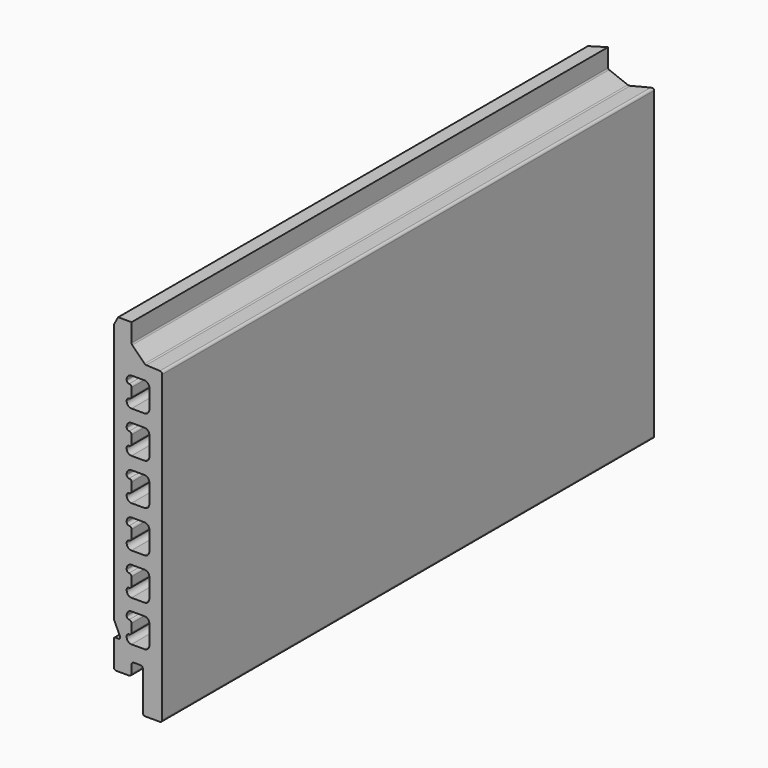
from build123d import *

# Parameters (mm, degrees)
F1_DEPTH      = 381
F3_DEPTH      = 711.2
F5_DEPTH      = 106.0997464
F5_DEPTH_BACK = 106.0997464


# Not quite as in the source:
# - ends of sketch curves that miss each other by under 0.0002 mm in the source are joined


with BuildPart() as f1:
    # F0 (on Front) → F1 (new body)
    with BuildSketch(Plane.XZ):
        with BuildLine():
            ThreePointArc((-14.9999680608, -58.9985104), (-14.96444377, -59.322873513), (-14.8595551032, -59.6318585804))
            Line((-14.8595551032, -59.6318585804), (-11.0988328608, -67.6967912))
            ThreePointArc((-11.0988328608, -67.6967912), (-11.1617050028, -68.655791158), (-12.004294, -69.1180454046))
            Line((-12.004294, -69.1180454046), (-14.0009118, -69.1180736))
            ThreePointArc((-14.0009118, -69.1180736), (-14.707352628, -69.410690972), (-14.99997, -70.1171318))
            Line((-14.99997, -70.1171318), (-14.99997, -85.599397))
            ThreePointArc((-14.99997, -85.599397), (-14.5606310505, -86.6600550505), (-13.499973, -87.099394))
            Line((-13.499973, -87.099394), (-5.5003446, -87.099394))
            ThreePointArc((-5.5003446, -87.099394), (-4.4396865495, -86.6600550505), (-4.0003476, -85.599397))
            Line((-4.0003476, -85.599397), (-4.0003476, -80.5996356))
            ThreePointArc((-4.0003476, -80.5996356), (-3.5610086505, -79.5389775495), (-2.5003506, -79.0996386))
            Line((-2.5003506, -79.0996386), (1.4838426, -79.0996386))
            ThreePointArc((1.4838426, -79.0996386), (2.5445365709, -79.5390134712), (2.9838395966, -80.5997372))
            Line((2.9838395966, -80.5997372), (2.98196, -104.5986224))
            ThreePointArc((2.98196, -104.5986224), (3.4212540492, -105.6593625482), (4.481957, -106.0987464))
            Line((4.481957, -106.0987464), (13.499973, -106.0987464))
            ThreePointArc((13.499973, -106.0987464), (14.5606310505, -105.6594074505), (14.99997, -104.5987494))
            Line((14.99997, -104.5987494), (14.99997, 83.7761342))
            ThreePointArc((14.99997, 83.7761342), (14.5844487053, 84.8124273268), (13.5680958768, 85.2745834897))
            Line((13.5680958768, 85.2745834897), (5.104384, 85.6592902))
            ThreePointArc((5.104384, 85.6592902), (4.5671403109, 85.7853117853), (4.1118233495, 86.0970797495))
            Line((4.1118233495, 86.0970797495), (-3.5610038, 93.7699166))
            ThreePointArc((-3.5610038, 93.7699166), (-3.8861671271, 94.2565457995), (-4.0003476, 94.8305698))
            Line((-4.0003476, 94.8305698), (-4.0003476, 106.0987464))
            Line((-4.0003476, 106.0987464), (-12.3105164, 106.0987464))
            Line((-12.3105164, 106.0987464), (-14.99997, 101.2086876))
            Line((-14.99997, 101.2086876), (-14.9999680608, -58.9985104))
        make_face()
    extrude(amount=F1_DEPTH)

    # F2 (on Front) → F3 (cut)
    with BuildSketch(Plane.XZ):
        with BuildLine():
            ThreePointArc((-5.49529, -31.195264), (-4.4346319495, -31.6346029495), (-3.995293, -32.695261))
            Line((-3.995293, -32.695261), (-3.995293, -37.695251))
            ThreePointArc((-3.995293, -37.695251), (-4.4346319495, -38.7559090505), (-5.49529, -39.195248))
            Line((-5.49529, -39.195248), (-5.499989, -39.195248))
            ThreePointArc((-5.499989, -39.195248), (-6.5606470505, -39.6345869495), (-6.999986, -40.695245))
            Line((-6.999986, -40.695245), (-6.999986, -41.195244))
            ThreePointArc((-6.999986, -41.195244), (-6.1213081009, -43.3165601009), (-3.999992, -44.195238))
            Line((-3.999992, -44.195238), (3.999992, -44.195238))
            ThreePointArc((3.999992, -44.195238), (6.1213081009, -43.3165601009), (6.999986, -41.195244))
            Line((6.999986, -41.195244), (6.999986, -29.195268))
            ThreePointArc((6.999986, -29.195268), (6.1213081009, -27.0739518991), (3.999992, -26.195274))
            Line((3.999992, -26.195274), (-3.999992, -26.195274))
            ThreePointArc((-3.999992, -26.195274), (-6.1213081009, -27.0739518991), (-6.999986, -29.195268))
            Line((-6.999986, -29.195268), (-6.999986, -29.695267))
            ThreePointArc((-6.999986, -29.695267), (-6.5606470505, -30.7559250505), (-5.499989, -31.195264))
            Line((-5.499989, -31.195264), (-5.49529, -31.195264))
        make_face()
        with BuildLine():
            ThreePointArc((-5.49529, -56.595264), (-4.4346319495, -57.0346029495), (-3.995293, -58.095261))
            Line((-3.995293, -58.095261), (-3.995293, -63.095251))
            ThreePointArc((-3.995293, -63.095251), (-4.4346319495, -64.1559090505), (-5.49529, -64.595248))
            Line((-5.49529, -64.595248), (-5.499989, -64.595248))
            ThreePointArc((-5.499989, -64.595248), (-6.5606470505, -65.0345869495), (-6.999986, -66.095245))
            Line((-6.999986, -66.095245), (-6.999986, -66.595244))
            ThreePointArc((-6.999986, -66.595244), (-6.1213081009, -68.7165601009), (-3.999992, -69.595238))
            Line((-3.999992, -69.595238), (0, -69.595238))
            Line((0, -69.595238), (3.999992, -69.595238))
            ThreePointArc((3.999992, -69.595238), (6.1213081009, -68.7165601009), (6.999986, -66.595244))
            Line((6.999986, -66.595244), (6.999986, -54.595268))
            ThreePointArc((6.999986, -54.595268), (6.1213081009, -52.4739518991), (3.999992, -51.595274))
            Line((3.999992, -51.595274), (-3.999992, -51.595274))
            ThreePointArc((-3.999992, -51.595274), (-6.1213081009, -52.4739518991), (-6.999986, -54.595268))
            Line((-6.999986, -54.595268), (-6.999986, -55.095267))
            ThreePointArc((-6.999986, -55.095267), (-6.5606470505, -56.1559250505), (-5.499989, -56.595264))
            Line((-5.499989, -56.595264), (-5.49529, -56.595264))
        make_face()
        with BuildLine():
            ThreePointArc((-5.49529, -5.3953664), (-4.4346319495, -5.8347053495), (-3.995293, -6.8953634))
            Line((-3.995293, -6.8953634), (-3.995293, -11.8953534))
            ThreePointArc((-3.995293, -11.8953534), (-4.4346319495, -12.9560114505), (-5.49529, -13.3953504))
            Line((-5.49529, -13.3953504), (-5.499989, -13.3953504))
            ThreePointArc((-5.499989, -13.3953504), (-6.5606470505, -13.8346893495), (-6.999986, -14.8953474))
            Line((-6.999986, -14.8953474), (-6.999986, -15.3953464))
            ThreePointArc((-6.999986, -15.3953464), (-6.1213081009, -17.5166625009), (-3.999992, -18.3953404))
            Line((-3.999992, -18.3953404), (3.999992, -18.3953404))
            ThreePointArc((3.999992, -18.3953404), (6.1213081009, -17.5166625009), (6.999986, -15.3953464))
            Line((6.999986, -15.3953464), (6.999986, -3.3953704))
            ThreePointArc((6.999986, -3.3953704), (6.1213081009, -1.2740542991), (3.999992, -0.3953764))
            Line((3.999992, -0.3953764), (-3.999992, -0.3953764))
            ThreePointArc((-3.999992, -0.3953764), (-6.1213081009, -1.2740542991), (-6.999986, -3.3953704))
            Line((-6.999986, -3.3953704), (-6.999986, -3.8953694))
            ThreePointArc((-6.999986, -3.8953694), (-6.5606470505, -4.9560274505), (-5.499989, -5.3953664))
            Line((-5.499989, -5.3953664), (-5.49529, -5.3953664))
        make_face()
        with BuildLine():
            Line((-5.499989, 20.4015086), (-5.49529, 20.4015086))
            ThreePointArc((-5.49529, 20.4015086), (-4.4346319495, 19.9621696505), (-3.995293, 18.9015116))
            Line((-3.995293, 18.9015116), (-3.995293, 13.9015216))
            ThreePointArc((-3.995293, 13.9015216), (-4.4346319495, 12.8408635495), (-5.49529, 12.4015246))
            Line((-5.49529, 12.4015246), (-5.499989, 12.4015246))
            ThreePointArc((-5.499989, 12.4015246), (-6.5606470505, 11.9621856505), (-6.999986, 10.9015276))
            Line((-6.999986, 10.9015276), (-6.999986, 10.4015286))
            ThreePointArc((-6.999986, 10.4015286), (-6.1213081009, 8.2802124991), (-3.999992, 7.4015346))
            Line((-3.999992, 7.4015346), (3.999992, 7.4015346))
            ThreePointArc((3.999992, 7.4015346), (6.1213081009, 8.2802124991), (6.999986, 10.4015286))
            Line((6.999986, 10.4015286), (6.999986, 22.4015046))
            ThreePointArc((6.999986, 22.4015046), (6.1213081009, 24.5228207009), (3.999992, 25.4014986))
            Line((3.999992, 25.4014986), (-3.999992, 25.4014986))
            ThreePointArc((-3.999992, 25.4014986), (-6.1213081009, 24.5228207009), (-6.999986, 22.4015046))
            Line((-6.999986, 22.4015046), (-6.999986, 21.9015056))
            ThreePointArc((-6.999986, 21.9015056), (-6.5606470505, 20.8408475495), (-5.499989, 20.4015086))
        make_face()
        with BuildLine():
            Line((-5.499989, 46.1983836), (-5.49529, 46.1983836))
            ThreePointArc((-5.49529, 46.1983836), (-4.4346319495, 45.7590446505), (-3.995293, 44.6983866))
            Line((-3.995293, 44.6983866), (-3.995293, 39.6983966))
            ThreePointArc((-3.995293, 39.6983966), (-4.4346319495, 38.6377385495), (-5.49529, 38.1983996))
            Line((-5.49529, 38.1983996), (-5.499989, 38.1983996))
            ThreePointArc((-5.499989, 38.1983996), (-6.5606470505, 37.7590606505), (-6.999986, 36.6984026))
            Line((-6.999986, 36.6984026), (-6.999986, 36.1984036))
            ThreePointArc((-6.999986, 36.1984036), (-6.1213081009, 34.0770874991), (-3.999992, 33.1984096))
            Line((-3.999992, 33.1984096), (3.999992, 33.1984096))
            ThreePointArc((3.999992, 33.1984096), (6.1213081009, 34.0770874991), (6.999986, 36.1984036))
            Line((6.999986, 36.1984036), (6.999986, 48.1983796))
            ThreePointArc((6.999986, 48.1983796), (6.1213081009, 50.3196957009), (3.999992, 51.1983736))
            Line((3.999992, 51.1983736), (-3.999992, 51.1983736))
            ThreePointArc((-3.999992, 51.1983736), (-6.1213081009, 50.3196957009), (-6.999986, 48.1983796))
            Line((-6.999986, 48.1983796), (-6.999986, 47.6983806))
            ThreePointArc((-6.999986, 47.6983806), (-6.5606470505, 46.6377225495), (-5.499989, 46.1983836))
        make_face()
        with BuildLine():
            Line((-5.499989, 71.9952586), (-5.49529, 71.9952586))
            ThreePointArc((-5.49529, 71.9952586), (-4.4346319495, 71.5559196505), (-3.995293, 70.4952616))
            Line((-3.995293, 70.4952616), (-3.995293, 65.4952716))
            ThreePointArc((-3.995293, 65.4952716), (-4.4346319495, 64.4346135495), (-5.49529, 63.9952746))
            Line((-5.49529, 63.9952746), (-5.499989, 63.9952746))
            ThreePointArc((-5.499989, 63.9952746), (-6.5606470505, 63.5559356505), (-6.999986, 62.4952776))
            Line((-6.999986, 62.4952776), (-6.999986, 61.9952786))
            ThreePointArc((-6.999986, 61.9952786), (-6.1213081009, 59.8739624991), (-3.999992, 58.9952846))
            Line((-3.999992, 58.9952846), (3.999992, 58.9952846))
            ThreePointArc((3.999992, 58.9952846), (6.1213081009, 59.8739624991), (6.999986, 61.9952786))
            Line((6.999986, 61.9952786), (6.999986, 73.9952546))
            ThreePointArc((6.999986, 73.9952546), (6.1213081009, 76.1165707009), (3.999992, 76.9952486))
            Line((3.999992, 76.9952486), (-3.999992, 76.9952486))
            ThreePointArc((-3.999992, 76.9952486), (-6.1213081009, 76.1165707009), (-6.999986, 73.9952546))
            Line((-6.999986, 73.9952546), (-6.999986, 73.4952556))
            ThreePointArc((-6.999986, 73.4952556), (-6.5606470505, 72.4345975495), (-5.499989, 71.9952586))
        make_face()
    extrude(amount=F3_DEPTH, mode=Mode.SUBTRACT)

    # F4 (on Top) → F5 (cut, two sides)
    with BuildSketch(Plane.XY) as f5_sk:
        Polygon((15.1597065851, 0), (-15.0980791077, 0), (-15.0980791077, -19.05), align=None)
    extrude(amount=-F5_DEPTH, mode=Mode.SUBTRACT)
    extrude(f5_sk.sketch, amount=F5_DEPTH_BACK, mode=Mode.SUBTRACT)


solid = f1.part
